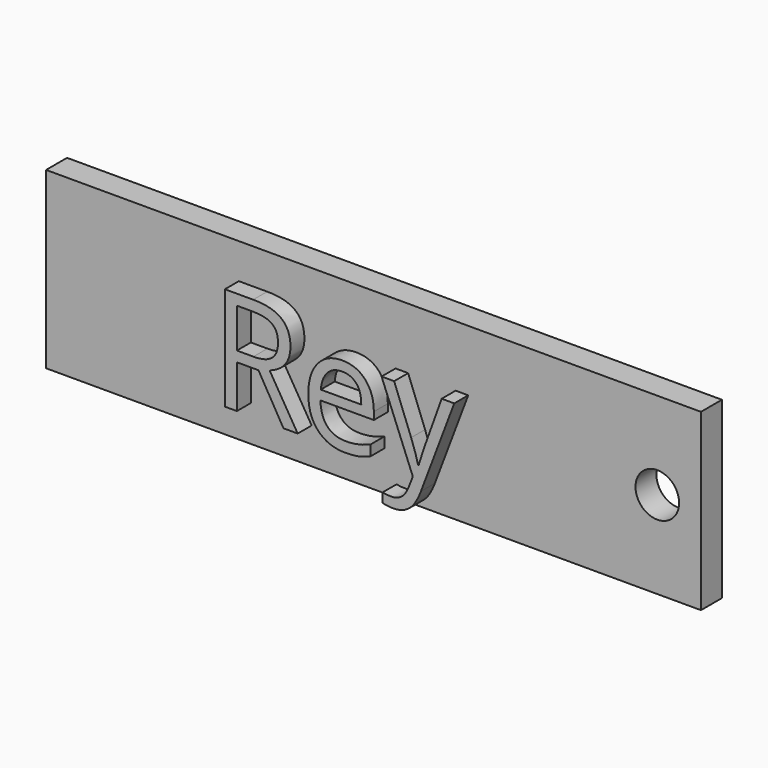
from build123d import *

# Parameters (mm, degrees)
F0_R         = 2.5
F1_DEPTH     = 3
F2_TEXT_SIZE = 16.5826621621
F3_DEPTH     = 2


# Not quite as in the source:
# - Text() gives the source's letters only with a copy of the font that has no kerning and outlines rounded to 1/6400 em; it was checked with that copy


with BuildPart() as f1:
    # F0 (on Front) → F1 (new body)
    with BuildSketch(Plane.XZ):
        Polygon((0, 0), (0, -2.9089373837), (0, -20), (75, -20), (75, 0), align=None)
        with Locations((70, -10)):
            Circle(F0_R, mode=Mode.SUBTRACT)
    extrude(amount=F1_DEPTH)

    # F2 (on face) → F3 (join)
    with BuildSketch(Plane.XZ.offset(3)):
        with Locations((20.4495959915, -15.87701682)):
            Text('Rey', F2_TEXT_SIZE, font='Open Sans', text_align=(TextAlign.LEFT, TextAlign.BOTTOM))
    extrude(amount=F3_DEPTH)


solid = f1.part
